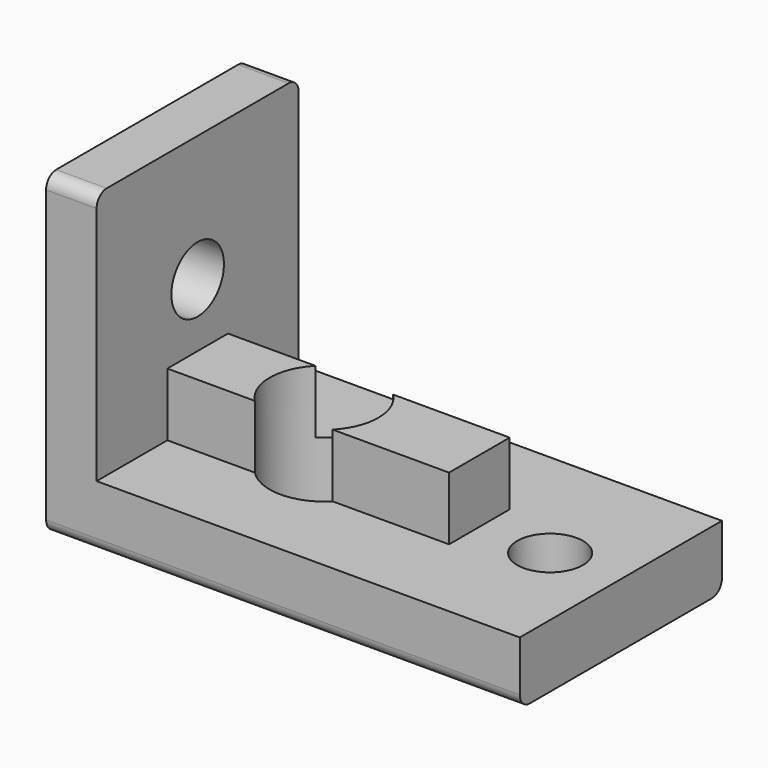
from build123d import *

# Parameters (mm, degrees)
F0_W      = 33.5
F0_H      = 20
F1_DEPTH  = 5
F2_W      = 33.5
F2_H      = 6
F3_DEPTH  = 5
F4_R      = 4.3
F5_DEPTH  = 25
F6_W      = 11.2
F6_H      = 6
F7_DEPTH  = 5
F8_R      = 2.6
F9_DEPTH  = 5
F10_R     = 2.6
F11_DEPTH = 4
F12_R     = 1


# Not quite as in the source:
# - a fillet or chamfer that OpenCascade refuses, or shapes differently, is made with other operations: its cross-section is extruded or revolved along the edge and cut away or added
# - a feature names something its author has since deleted; it is built from what else it names


with BuildPart() as f1:
    # F0 (on Top) → F1 (new body)
    with BuildSketch(Plane.XY):
        with Locations((16.75, 0)):
            Rectangle(F0_W, F0_H)
    extrude(amount=F1_DEPTH)

    # F2 (on face) → F3 (join)
    with BuildSketch(Plane.XY.offset(5)):
        with Locations((16.75, 0)):
            Rectangle(F2_W, F2_H)
    extrude(amount=F3_DEPTH)

    # F4 (on face) → F5 (cut)
    with BuildSketch(Plane.XY.offset(10)):
        with Locations((10, 0)):
            Circle(F4_R)
    extrude(amount=-F5_DEPTH, mode=Mode.SUBTRACT)

    # F6 (on face) → F7 (cut, through all)
    with BuildSketch(Plane.XY.offset(10)):
        with Locations((27.9, 0)):
            Rectangle(F6_W, F6_H)
    extrude(amount=-F7_DEPTH, mode=Mode.SUBTRACT)

    # F8 (on face) → F9 (cut, through all)
    with BuildSketch(Plane.XY.offset(5)):
        with Locations((27.9, 0)):
            Circle(F8_R)
    extrude(amount=-F9_DEPTH, mode=Mode.SUBTRACT)

    # F10 (on face) → F11 (join)
    with BuildSketch(Plane(origin=(0, 0, 0), x_dir=(0, -1, 0), z_dir=(-1, 0, 0))):
        Polygon((-10, 25), (-10, 5), (-3, 5), (-3, 10), (3, 10), (3, 5), (10, 5), (10, 25), align=None)
        with Locations((0, 15)):
            Circle(F10_R, mode=Mode.SUBTRACT)
        Polygon((-10, 5), (-10, 0), (10, 0), (10, 5), (3, 5), (3, 10), (-3, 10), (-3, 5), align=None)
    extrude(amount=F11_DEPTH)

    # F12
    f12_edges = [f1.edges().sort_by_distance(p)[0] for p in [
        (-2, -10, 25),
        (-2, 10, 25),
        (14.75, -10, 0),
        (14.75, 10, 0),
    ]]
    fillet(f12_edges, radius=F12_R)

    # F13: chamfer of 0.5 x 0.2886751346 on 1 edges, made by hand

    # F13_s1 → F13_t2 (revolve, cut)
    with BuildSketch(Plane.XZ):
        Polygon((14.5886751346, 0), (14.3, 0.5), (14.3, 0), align=None)
    revolve(axis=Axis((10, 0, 0), (0, 0, 1)), mode=Mode.SUBTRACT)


solid = f1.part
